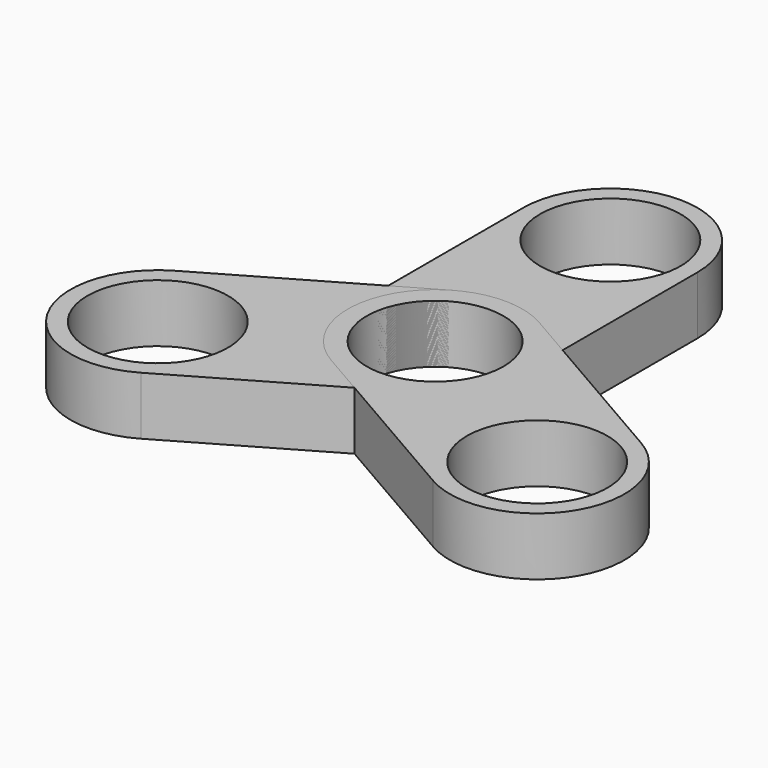
from build123d import *

# Parameters (mm, degrees)
F1_DEPTH        = 7
F1_COPIES_COUNT = 3


# Not quite as in the source:
# - a feature of the source that left no trace in its solid (it failed there, or was rolled back) is left out
# - a pattern or mirror of a feature is missing from the dataset's text; its kind, count and spacing are read off the source's solid


with BuildPart() as f1:
    # F0 (on Top) → F1 (new body)
    with BuildSketch(Plane.XY):
        with BuildLine():
            Line((27.8392881155, -14.3839418888), (27.8392881155, 12.004762888))
            ThreePointArc((27.8392881155, 12.004762888), (17.329832539, 1.4953073114), (6.8203769624, 12.004762888))
            Line((6.8203769624, 12.004762888), (6.8203769624, -14.3839418888))
            ThreePointArc((6.8203769624, -14.3839418888), (17.329832539, -3.8744863123), (27.8392881155, -14.3839418888))
        make_face()
        with BuildLine():
            ThreePointArc((8.8624665908, 12.004762888), (17.329832539, 20.4721288361), (25.7971984871, 12.004762888))
            Line((25.7971984871, 12.004762888), (27.8392881155, 12.004762888))
            ThreePointArc((27.8392881155, 12.004762888), (17.329832539, 22.5142184645), (6.8203769624, 12.004762888))
            Line((6.8203769624, 12.004762888), (8.8624665908, 12.004762888))
        make_face()
        with BuildLine():
            Line((27.8392881155, 12.004762888), (25.7971984871, 12.004762888))
            ThreePointArc((25.7971984871, 12.004762888), (17.329832539, 3.5373969398), (8.8624665908, 12.004762888))
            Line((8.8624665908, 12.004762888), (6.8203769624, 12.004762888))
            ThreePointArc((6.8203769624, 12.004762888), (17.329832539, 1.4953073114), (27.8392881155, 12.004762888))
        make_face()
        with BuildLine():
            Line((25.5679596325, -14.3839418888), (27.8392881155, -14.3839418888))
            ThreePointArc((27.8392881155, -14.3839418888), (17.329832539, -3.8744863123), (6.8203769624, -14.3839418888))
            Line((6.8203769624, -14.3839418888), (9.0917054454, -14.3839418888))
            ThreePointArc((9.0917054454, -14.3839418888), (17.329832539, -6.1458147953), (25.5679596325, -14.3839418888))
        make_face()
        with BuildLine():
            ThreePointArc((6.8203769624, -14.3839418888), (17.329832539, -24.8933974653), (27.8392881155, -14.3839418888))
            Line((27.8392881155, -14.3839418888), (25.5679596325, -14.3839418888))
            ThreePointArc((25.5679596325, -14.3839418888), (17.329832539, -22.6220689824), (9.0917054454, -14.3839418888))
            Line((9.0917054454, -14.3839418888), (6.8203769624, -14.3839418888))
        make_face()
    extrude(amount=F1_DEPTH)


with BuildPart() as f1_copies_1:
    # F1_copies: instance of F1
    add(f1.part.rotate(Axis((17.329833, -14.383942, 0), (0, 0, 1)), 1 * 360 / F1_COPIES_COUNT))


with BuildPart() as f1_copies_2:
    # F1_copies: instance of F1
    add(f1.part.rotate(Axis((17.329833, -14.383942, 0), (0, 0, 1)), 2 * 360 / F1_COPIES_COUNT))


solid = Compound([f1.part, f1_copies_1.part, f1_copies_2.part])
